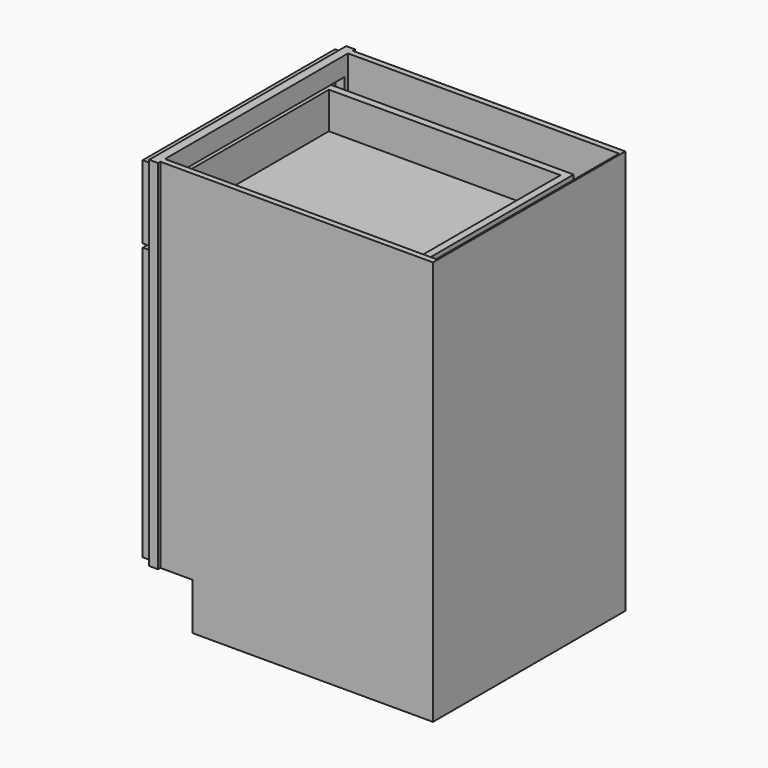
from build123d import *

# Parameters (mm, degrees)
F0_W          = 609.6
F0_H          = 876.3
F1_DEPTH      = 533.4
F2_W          = 88.9
F2_H          = 101.6
F3_DEPTH      = 533.401
F4_W          = 476.562295082
F4_H          = 692.15
F5_DEPTH      = 19.05
F6_W          = 590.55
F6_H          = 6.35
F7_DEPTH      = 876.301
F8_W          = 587.375
F8_H          = 495.3
F9_DEPTH      = 733.425
F10_W         = 476.562295082
F10_H         = 41.275
F11_DEPTH     = 19.05
F12_W         = 520.7
F12_H         = 590.5627
F12_W_2       = 406.4
F12_H_2       = 476.2627
F13_DEPTH     = 19.05
F14_W         = 6.35
F14_H         = 406.4
F15_DEPTH     = 476.2627
F16_SIZE      = 3.175
F17_W         = 520.7
F17_H         = 158.75
F17_W_2       = 406.4
F17_H_2       = 82.55
F18_DEPTH     = 19.05
F19_W         = 6.35
F19_H         = 406.4
F20_DEPTH     = 82.55
F21_SIZE      = 3.175
F22_W         = 504.825
F22_H         = 495.3
F23_DEPTH     = 101.6
F24_W         = 431.8
F24_H         = 95.25
F25_DEPTH     = 533.4
F26_T         = 15.875
F26_T3_DEPTH  = 37.249261314
F26_T5_DEPTH  = 37.249261314
F26_T7_DEPTH  = 37.249261314
F26_T9_DEPTH  = 37.249261314
F26_T11_DEPTH = 36.5125
F26_T13_DEPTH = 438.15
F26_T15_DEPTH = 114.3
F26_T17_DEPTH = 127
F26_T19_DEPTH = 463.55
F26_T21_DEPTH = 111.125
F26_T23_DEPTH = 36.5125


# Not quite as in the source:
# - a shell that OpenCascade refuses in one call is made with other operations: the cavity is built on its own and cut out


with BuildPart() as f1:
    # F0 (on Front) → F1 (new body)
    with BuildSketch(Plane.XZ):
        Rectangle(F0_W, F0_H)
    extrude(amount=-F1_DEPTH)

    # F2 (on face) → F3 (cut, through all)
    with BuildSketch(Plane.XZ):
        with Locations((-260.35, -387.35)):
            Rectangle(F2_W, F2_H)
    extrude(amount=-F3_DEPTH, mode=Mode.SUBTRACT)

    # F4 (on face) → F5 (cut)
    with BuildSketch(Plane(origin=(-304.8, 0, 0), x_dir=(0, -1, 0), z_dir=(-1, 0, 0))):
        with Locations((-266.7, 50.8)):
            Rectangle(F4_W, F4_H)
    extrude(amount=-F5_DEPTH, mode=Mode.SUBTRACT)

    # F6 (on face) → F7 (cut, through all)
    with BuildSketch(Plane.XY.offset(438.15)):
        with Locations((9.525, 530.225)):
            Rectangle(F6_W, F6_H)
        with Locations((9.525, 3.175)):
            Rectangle(F6_W, F6_H)
    extrude(amount=-F7_DEPTH, mode=Mode.SUBTRACT)

    # F8 (on face) → F9 (cut, through all)
    with BuildSketch(Plane.XY.offset(438.15)):
        with Locations((7.9375, 266.7)):
            Rectangle(F8_W, F8_H)
    extrude(amount=-F9_DEPTH, mode=Mode.SUBTRACT)

    # F10 (on face) → F11 (join, through all)
    with BuildSketch(Plane(origin=(-304.8, 0, 0), x_dir=(0, -1, 0), z_dir=(-1, 0, 0))):
        with Locations((-266.7, 265.1125)):
            Rectangle(F10_W, F10_H)
    extrude(amount=-F11_DEPTH)

    # F22 (on face) → F23 (cut)
    with BuildSketch(Plane(origin=(0, 0, -438.15), x_dir=(1, 0, 0), z_dir=(0, 0, -1))):
        with Locations((49.2125, -266.7)):
            Rectangle(F22_W, F22_H)
    extrude(amount=-F23_DEPTH, mode=Mode.SUBTRACT)


with BuildPart() as f13:
    # F12 (on face) → F13 (new body)
    with BuildSketch(Plane(origin=(-304.8, 0, 0), x_dir=(0, -1, 0), z_dir=(-1, 0, 0))):
        with Locations((-266.7, -33.33115)):
            Rectangle(F12_W, F12_H)
        with Locations((-266.7, -33.33115)):
            Rectangle(F12_W_2, F12_H_2, mode=Mode.SUBTRACT)
    extrude(amount=F13_DEPTH)

    # F14 (on face) → F15 (join, through all)
    with BuildSketch(Plane.XY.offset(-271.4625)):
        with Locations((-312.7375, 266.7)):
            Rectangle(F14_W, F14_H)
    extrude(amount=F15_DEPTH)

    # F16
    f16_edges = [f13.edges().sort_by_distance(p)[0] for p in [
        (-323.85, 469.9, -33.33115),
        (-323.85, 266.7, -271.4625),
        (-323.85, 63.5, -33.33115),
        (-323.85, 266.7, 204.8002),
    ]]
    chamfer(f16_edges, length=F16_SIZE)


with BuildPart() as f18:
    # F17 (on face) → F18 (new body)
    with BuildSketch(Plane(origin=(-304.8, 0, 0), x_dir=(0, -1, 0), z_dir=(-1, 0, 0))):
        with Locations((-266.7, 349.25)):
            Rectangle(F17_W, F17_H)
        with Locations((-266.7, 349.25)):
            Rectangle(F17_W_2, F17_H_2, mode=Mode.SUBTRACT)
    extrude(amount=F18_DEPTH)

    # F19 (on face) → F20 (join, through all)
    with BuildSketch(Plane.XY.offset(307.975)):
        with Locations((-312.7375, 266.7)):
            Rectangle(F19_W, F19_H)
    extrude(amount=F20_DEPTH)

    # F21
    f21_edges = [f18.edges().sort_by_distance(p)[0] for p in [
        (-323.85, 266.7, 307.975),
        (-323.85, 469.9, 349.25),
        (-323.85, 266.7, 390.525),
        (-323.85, 63.5, 349.25),
    ]]
    chamfer(f21_edges, length=F21_SIZE)

    # F24 (on face) → F25 (join)
    with BuildSketch(Plane.YZ.offset(-304.8)):
        with Locations((266.7, 339.725)):
            Rectangle(F24_W, F24_H)
    extrude(amount=F25_DEPTH)

    # F26: shell of thickness 15.875, made by hand


with BuildPart() as f26_core1:
    # F26_t2: copy of F18
    add(f18.part)

    # the walls: a layer under each face that stays
    f26_faces = [f26_core1.faces().sort_by_distance(p)[0] for p in [
        (-323.85, 440.2666666667, 296.3333333333),
        (-322.2625, 266.7, 306.3875),
        (-322.2625, 61.9125, 349.25),
        (-322.2625, 471.4875, 349.25),
        (-322.2625, 266.7, 392.1125),
        (-314.325, 266.7, 428.625),
        (-314.325, 527.05, 349.25),
        (-314.325, 266.7, 269.875),
        (-314.325, 6.35, 349.25),
        (-318.29375, 266.7, 307.975),
        (-318.29375, 63.5, 349.25),
        (-318.29375, 469.9, 349.25),
        (-318.29375, 266.7, 390.525),
        (-304.8, 440.2666666667, 402.1666666667),
        (-315.9125, 266.7, 349.25),
        (-38.1, 482.6, 339.725),
        (-38.1, 266.7, 292.1),
        (-38.1, 50.8, 339.725),
        (-307.18125, 63.5, 349.25),
        (-307.18125, 266.7, 390.525),
        (-307.18125, 469.9, 349.25),
        (-304.8, 266.7, 347.6625),
        (228.6, 266.7, 339.725),
        (-307.18125, 266.7, 307.975),
        (-309.5625, 266.7, 349.25),
    ]]
    thicken(f26_faces, amount=-F26_T, mode=Mode.SUBTRACT)

    # F26_s4 → F26_t3 (cut)
    with BuildSketch(Plane(origin=(4.5928978099, 4.5928978099, 4.5928978099), x_dir=(-0.7071067812, 0.7071067812, 0), z_dir=(0.5773502692, 0.5773502692, 0.5773502692))):
        Polygon((271.8908726623, 356.5892701441), (263.7152476623, 342.7036353262), (255.7777476623, 347.2863530879), (255.7777476623, 356.4517886113), align=None)
    extrude(amount=F26_T3_DEPTH, mode=Mode.SUBTRACT)

    # F26_s6 → F26_t5 (cut)
    with BuildSketch(Plane(origin=(-173.2071021901, 173.2071021901, -173.2071021901), x_dir=(0.7071067812, 0.7071067812, 0), z_dir=(0.5773502692, -0.5773502692, 0.5773502692))):
        Polygon((105.2798844226, 574.3489082775), (113.4555094226, 560.4632734596), (121.3930094226, 565.0459912213), (121.3930094226, 574.2114267447), align=None)
    extrude(amount=F26_T5_DEPTH, mode=Mode.SUBTRACT)

    # F26_s8 → F26_t7 (cut)
    with BuildSketch(Plane(origin=(-228.2404355234, -228.2404355234, 228.2404355234), x_dir=(-0.7071067812, 0.7071067812, 0), z_dir=(0.5773502692, 0.5773502692, -0.5773502692))):
        Polygon((271.8908726623, 213.7335916339), (255.7777476623, 213.8710731668), (255.7777476623, 223.0365086901), (263.7152476623, 227.6192264518), align=None)
    extrude(amount=F26_T7_DEPTH, mode=Mode.SUBTRACT)

    # F26_s10 → F26_t9 (cut)
    with BuildSketch(Plane(origin=(-406.0404355234, 406.0404355234, 406.0404355234), x_dir=(0.7071067812, 0.7071067812, 0), z_dir=(0.5773502692, -0.5773502692, -0.5773502692))):
        Polygon((105.2798844226, -4.0260464995), (121.3930094226, -3.8885649667), (121.3930094226, 5.2768705567), (113.4555094226, 9.8595883184), align=None)
    extrude(amount=F26_T9_DEPTH, mode=Mode.SUBTRACT)

    # F26_s12 → F26_t11 (cut)
    with BuildSketch(Plane.YZ.offset(-336.55)):
        Polygon((469.74125, 308.13375), (469.9, 292.1), (485.775, 292.1), (485.775, 307.975), align=None)
        Polygon((63.65875, 308.13375), (63.5, 292.1), (47.625, 292.1), (47.625, 307.975), align=None)
        Polygon((63.65875, 390.36625), (47.625, 390.525), (47.625, 406.4), (63.5, 406.4), align=None)
        Polygon((469.74125, 390.36625), (485.775, 390.525), (485.775, 406.4), (469.9, 406.4), align=None)
    extrude(amount=F26_T11_DEPTH, mode=Mode.SUBTRACT)

    # F26_s14 → F26_t13 (cut)
    with BuildSketch(Plane.XZ.offset(-485.775)):
        Polygon((-316.07125, 308.13375), (-315.9125, 292.1), (-300.0375, 292.1), (-300.0375, 307.975), align=None)
        Polygon((-316.07125, 390.36625), (-315.9125, 406.4), (-300.0375, 406.4), (-300.0375, 390.525), align=None)
        Polygon((-309.40375, 390.36625), (-309.5625, 406.4), (-325.4375, 406.4), (-325.4375, 390.525), align=None)
        Polygon((-304.95875, 308.13375), (-288.925, 307.975), (-288.925, 292.1), (-304.8, 292.1), align=None)
        Polygon((-309.40375, 308.13375), (-309.5625, 292.1), (-325.4375, 292.1), (-325.4375, 307.975), align=None)
    extrude(amount=F26_T13_DEPTH, mode=Mode.SUBTRACT)

    # F26_s16 → F26_t15 (cut)
    with BuildSketch(Plane.XY.offset(292.1)):
        Polygon((-316.07125, 63.65875), (-315.9125, 47.625), (-300.0375, 47.625), (-300.0375, 63.5), align=None)
        Polygon((-316.07125, 469.74125), (-315.9125, 485.775), (-300.0375, 485.775), (-300.0375, 469.9), align=None)
        Polygon((-309.40375, 63.65875), (-309.5625, 47.625), (-325.4375, 47.625), (-325.4375, 63.5), align=None)
        Polygon((-309.40375, 469.74125), (-309.5625, 485.775), (-325.4375, 485.775), (-325.4375, 469.9), align=None)
    extrude(amount=F26_T15_DEPTH, mode=Mode.SUBTRACT)

    # F26_s18 → F26_t17 (cut)
    with BuildSketch(Plane.XY.offset(276.225)):
        Polygon((-304.64125, 482.75875), (-320.675, 482.6), (-320.675, 466.725), (-304.8, 466.725), align=None)
        Polygon((-304.64125, 50.64125), (-320.675, 50.8), (-320.675, 66.675), (-304.8, 66.675), align=None)
    extrude(amount=F26_T17_DEPTH, mode=Mode.SUBTRACT)

    # F26_s20 → F26_t19 (cut)
    with BuildSketch(Plane.XZ.offset(-498.475)):
        Polygon((-304.64125, 291.94125), (-320.675, 292.1), (-320.675, 307.975), (-304.8, 307.975), align=None)
    extrude(amount=F26_T19_DEPTH, mode=Mode.SUBTRACT)

    # F26_s22 → F26_t21 (cut)
    with BuildSketch(Plane.XY.offset(292.1)):
        Polygon((-304.95875, 63.65875), (-304.8, 47.625), (-288.925, 47.625), (-288.925, 63.5), align=None)
        Polygon((-304.95875, 469.74125), (-304.8, 485.775), (-288.925, 485.775), (-288.925, 469.9), align=None)
    extrude(amount=F26_T21_DEPTH, mode=Mode.SUBTRACT)

    # F26_s24 → F26_t23 (cut)
    with BuildSketch(Plane.YZ.offset(-325.4375)):
        Polygon((63.65875, 308.13375), (47.625, 307.975), (47.625, 292.1), (63.5, 292.1), align=None)
        Polygon((63.65875, 390.36625), (47.625, 390.525), (47.625, 406.4), (63.5, 406.4), align=None)
        Polygon((469.74125, 390.36625), (469.9, 406.4), (485.775, 406.4), (485.775, 390.525), align=None)
        Polygon((469.74125, 308.13375), (485.775, 307.975), (485.775, 292.1), (469.9, 292.1), align=None)
    extrude(amount=F26_T23_DEPTH, mode=Mode.SUBTRACT)


with BuildPart() as f18_1:
    add(f18.part)

    # what is left inside the walls is the cavity
    f26_cavity = [f26_core1.part.solids().sort_by_distance(p)[0] for p in [
        (45.508333, 266.7, 308.13375),
    ]]
    add(f26_cavity, mode=Mode.SUBTRACT)


solid = Compound([f1.part, f13.part, f18_1.part])
